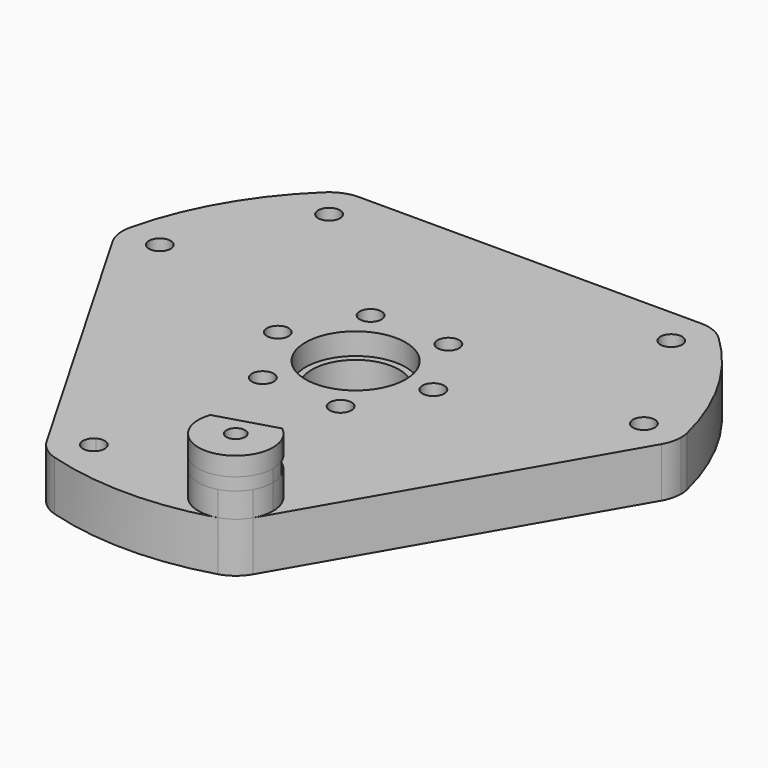
from build123d import *

# Parameters (mm, degrees)
F0_R     = 1.75
F0_R_2   = 8.05
F0_R_3   = 1.5
F0_R_4   = 7
F1_DEPTH = 8
F2_DEPTH = 3.5
F3_DEPTH = 4
F5_DEPTH = 2
F7_DEPTH = 3


# Not quite as in the source:
# - a feature names something its author has since deleted; it is built from what else it names


with BuildPart() as f1:
    # F0 (on Top) → F1 (new body)
    with BuildSketch(Plane.XY):
        with BuildLine():
            ThreePointArc((-32.9057647469, 9.2920110558), (-33.7096123242, 6.2920110558), (-35.9057647469, 4.0958586331))
            Line((-35.9057647469, 4.0958586331), (-14.4057647469, -33.1432337296))
            ThreePointArc((-14.4057647469, -33.1432337296), (-8.4057647469, -33.1432337296), (-5.4057647469, -38.3393861523))
            ThreePointArc((-5.4057647469, -38.3393861523), (-7.8186481903, -43.1490217736), (-13.1166296833, -44.0902940084))
            ThreePointArc((-13.1166296833, -44.0902940084), (-2.42e-07, -46), (13.1166292194, -44.0902941464))
            ThreePointArc((13.1166292194, -44.0902941464), (6.5961292703, -34.7522694018), (17.4057647469, -38.3393861523))
            ThreePointArc((17.4057647469, -38.3393861523), (17.2013197046, -39.892300423), (16.6019171696, -41.3393861523))
            Line((16.6019171696, -41.3393861523), (44.1019171696, 6.2920110558))
            ThreePointArc((44.1019171696, 6.2920110558), (32.9683642938, 10.1564622456), (44.7416293579, 10.685813137))
            ThreePointArc((44.7416293579, 10.685813137), (39.8371685393, 23.0000000602), (31.6250002147, 33.4044811578))
            ThreePointArc((31.6250002147, 33.4044811578), (33.0113519797, 31.4190832059), (33.5, 29.0473750966))
            ThreePointArc((33.5, 29.0473750966), (27.5, 23.0473750966), (21.5, 29.0473750966))
            Line((21.5, 29.0473750966), (-21.5, 29.0473750966))
            ThreePointArc((-21.5, 29.0473750966), (-29.8717083356, 23.5360232142), (-31.624999857, 33.4044814964))
            ThreePointArc((-31.624999857, 33.4044814964), (-39.837168539, 23.0000000607), (-44.7416294721, 10.6858126589))
            ThreePointArc((-44.7416294721, 10.6858126589), (-38.2040484051, 15.2508359547), (-32.9057647469, 9.2920110558))
        make_face()
        with Locations((-6.25, -10.8253175473)):
            Circle(F0_R, mode=Mode.SUBTRACT)
        with Locations((6.25, -10.8253175473)):
            Circle(F0_R, mode=Mode.SUBTRACT)
        with Locations((-12.5, 0)):
            Circle(F0_R, mode=Mode.SUBTRACT)
        with Locations((-6.25, 10.8253175473)):
            Circle(F0_R, mode=Mode.SUBTRACT)
        Circle(F0_R_2, mode=Mode.SUBTRACT)
        with Locations((6.25, 10.8253175473)):
            Circle(F0_R, mode=Mode.SUBTRACT)
        with Locations((12.5, 0)):
            Circle(F0_R, mode=Mode.SUBTRACT)
        with BuildLine():
            Line((27.5, 35.0473750966), (-27.5, 35.0473750966))
            ThreePointArc((-27.5, 35.0473750966), (-23.2573593129, 33.2900157837), (-21.5, 29.0473750966))
            Line((-21.5, 29.0473750966), (21.5, 29.0473750966))
            ThreePointArc((21.5, 29.0473750966), (23.2573593129, 33.2900157837), (27.5, 35.0473750966))
        make_face()
        with BuildLine():
            ThreePointArc((-27.5, 35.0473750966), (-29.7200632424, 34.6215404331), (-31.624999857, 33.4044814964))
            ThreePointArc((-31.624999857, 33.4044814964), (-29.8717083356, 23.5360232142), (-21.5, 29.0473750966))
            ThreePointArc((-21.5, 29.0473750966), (-23.2573593129, 33.2900157837), (-27.5, 35.0473750966))
        make_face()
        with Locations((-27.5, 29.0473750966)):
            Circle(F0_R, mode=Mode.SUBTRACT)
        with BuildLine():
            ThreePointArc((33.5, 29.0473750966), (33.0113519797, 31.4190832059), (31.6250002147, 33.4044811578))
            ThreePointArc((31.6250002147, 33.4044811578), (29.7200634712, 34.621540342), (27.5, 35.0473750966))
            ThreePointArc((27.5, 35.0473750966), (23.2573593129, 33.2900157837), (21.5, 29.0473750966))
            ThreePointArc((21.5, 29.0473750966), (27.5, 23.0473750966), (33.5, 29.0473750966))
        make_face()
        with BuildLine():
            ThreePointArc((29.25, 29.0473750966), (27.5, 27.2973750966), (25.75, 29.0473750966))
            ThreePointArc((25.75, 29.0473750966), (27.5, 30.7973750966), (29.25, 29.0473750966))
        make_face(mode=Mode.SUBTRACT)
        with BuildLine():
            ThreePointArc((44.9057647469, 9.2920110558), (44.864589617, 9.9937276417), (44.7416293579, 10.685813137))
            ThreePointArc((44.7416293579, 10.685813137), (32.9683642938, 10.1564622456), (44.1019171696, 6.2920110558))
            ThreePointArc((44.1019171696, 6.2920110558), (44.7013197046, 7.7390967852), (44.9057647469, 9.2920110558))
        make_face()
        with Locations((38.9057647469, 9.2920110558)):
            Circle(F0_R, mode=Mode.SUBTRACT)
        with BuildLine():
            ThreePointArc((17.4057647469, -38.3393861523), (6.5961292703, -34.7522694018), (13.1166292194, -44.0902941464))
            ThreePointArc((13.1166292194, -44.0902941464), (15.1231017367, -43.049100125), (16.6019171696, -41.3393861523))
            ThreePointArc((16.6019171696, -41.3393861523), (17.2013197046, -39.892300423), (17.4057647469, -38.3393861523))
        make_face()
        with Locations((11.4057647469, -38.3393861523)):
            Circle(F0_R_3, mode=Mode.SUBTRACT)
        with BuildLine():
            ThreePointArc((-5.4057647469, -38.3393861523), (-8.4057647469, -33.1432337296), (-14.4057647469, -33.1432337296))
            ThreePointArc((-14.4057647469, -33.1432337296), (-17.2013197046, -36.7864718817), (-16.6019171696, -41.3393861523))
            ThreePointArc((-16.6019171696, -41.3393861523), (-15.1231019266, -43.0490999751), (-13.1166296833, -44.0902940084))
            ThreePointArc((-13.1166296833, -44.0902940084), (-7.8186481903, -43.1490217736), (-5.4057647469, -38.3393861523))
        make_face()
        with BuildLine():
            ThreePointArc((-9.6557647469, -38.3393861523), (-12.2807647469, -39.854930609), (-12.2807647469, -36.8238416957))
            ThreePointArc((-12.2807647469, -36.8238416957), (-10.5307647469, -36.8238416957), (-9.6557647469, -38.3393861523))
        make_face(mode=Mode.SUBTRACT)
        with BuildLine():
            Line((-14.4057647469, -33.1432337296), (-35.9057647469, 4.0958586331))
            ThreePointArc((-35.9057647469, 4.0958586331), (-40.4586790175, 3.4964560981), (-44.1019171696, 6.2920110558))
            Line((-44.1019171696, 6.2920110558), (-16.6019171696, -41.3393861523))
            ThreePointArc((-16.6019171696, -41.3393861523), (-17.2013197046, -36.7864718817), (-14.4057647469, -33.1432337296))
        make_face()
        with BuildLine():
            ThreePointArc((-44.1019171696, 6.2920110558), (-40.4586790175, 3.4964560981), (-35.9057647469, 4.0958586331))
            ThreePointArc((-35.9057647469, 4.0958586331), (-33.7096123242, 6.2920110558), (-32.9057647469, 9.2920110558))
            ThreePointArc((-32.9057647469, 9.2920110558), (-38.2040484051, 15.2508359547), (-44.7416294721, 10.6858126589))
            ThreePointArc((-44.7416294721, 10.6858126589), (-44.8431651646, 8.4275596228), (-44.1019171696, 6.2920110558))
        make_face()
        with BuildLine():
            ThreePointArc((-38.0307647469, 7.7764665992), (-40.4213092035, 10.1670110558), (-37.1557647469, 9.2920110558))
            ThreePointArc((-37.1557647469, 9.2920110558), (-37.3902202902, 8.4170110558), (-38.0307647469, 7.7764665992))
        make_face(mode=Mode.SUBTRACT)
        Circle(F0_R_2)
        Circle(F0_R_4, mode=Mode.SUBTRACT)
    extrude(amount=-F1_DEPTH)

    # F0 (on Top) → F2 (cut)
    with BuildSketch(Plane.XY):
        Circle(F0_R_2)
        Circle(F0_R_4, mode=Mode.SUBTRACT)
    extrude(amount=-F2_DEPTH, mode=Mode.SUBTRACT)


with BuildPart() as f3:
    # F0 (on Top) → F3 (new body)
    with BuildSketch(Plane.XY):
        with BuildLine():
            ThreePointArc((17.4057647469, -38.3393861523), (6.5961292703, -34.7522694018), (13.1166292194, -44.0902941464))
            ThreePointArc((13.1166292194, -44.0902941464), (15.1231017367, -43.049100125), (16.6019171696, -41.3393861523))
            ThreePointArc((16.6019171696, -41.3393861523), (17.2013197046, -39.892300423), (17.4057647469, -38.3393861523))
        make_face()
        with Locations((11.4057647469, -38.3393861523)):
            Circle(F0_R_3, mode=Mode.SUBTRACT)
    extrude(amount=F3_DEPTH)

    # F4 (on face) → F5 (join)
    with BuildSketch(Plane.XY.offset(4)):
        with BuildLine():
            ThreePointArc((9.9602708355, -38.7400697584), (7.7638146886, -39.2393065877), (5.5427392086, -39.6141141775))
            ThreePointArc((5.5427392086, -39.6141141775), (12.0467978079, -44.3050442564), (17.4057647469, -38.3393861523))
            ThreePointArc((17.4057647469, -38.3393861523), (17.3065432967, -37.2527341815), (17.0121605783, -36.2020219388))
            ThreePointArc((17.0121605783, -36.2020219388), (14.947389292, -37.1022311102), (12.8352193016, -37.8847877845))
            ThreePointArc((12.8352193016, -37.8847877845), (12.8880234679, -38.1093664054), (12.9057647469, -38.3393861523))
            ThreePointArc((12.9057647469, -38.3393861523), (11.607951706, -39.8256971674), (9.9602708355, -38.7400697584))
        make_face()
    extrude(amount=F5_DEPTH)

    # F6 (on face) → F7 (join)
    with BuildSketch(Plane.XY.offset(6)):
        with BuildLine():
            ThreePointArc((5.5427392086, -39.6141141775), (13.1166294589, -44.0902940752), (17.0121605783, -36.2020219388))
            ThreePointArc((17.0121605783, -36.2020219388), (14.947389292, -37.1022311102), (12.8352193016, -37.8847877845))
            ThreePointArc((12.8352193016, -37.8847877845), (12.8880234679, -38.1093664054), (12.9057647469, -38.3393861523))
            ThreePointArc((12.9057647469, -38.3393861523), (11.607951706, -39.8256971674), (9.9602708355, -38.7400697584))
            ThreePointArc((9.9602708355, -38.7400697584), (7.7638146886, -39.2393065877), (5.5427392086, -39.6141141775))
        make_face()
        with BuildLine():
            ThreePointArc((12.8352193016, -37.8847877845), (14.947389292, -37.1022311102), (17.0121605783, -36.2020219388))
            ThreePointArc((17.0121605783, -36.2020219388), (16.2239290423, -34.7637333696), (15.0756758433, -33.5926238301))
            Line((15.0756758433, -33.5926238301), (5.737994077, -36.3705348035))
            ThreePointArc((5.737994077, -36.3705348035), (5.4166064515, -37.9788547209), (5.5427392086, -39.6141141775))
            ThreePointArc((5.5427392086, -39.6141141775), (7.7638146886, -39.2393065877), (9.9602708355, -38.7400697584))
            ThreePointArc((9.9602708355, -38.7400697584), (10.9780485689, -36.9016591716), (12.8352193016, -37.8847877845))
        make_face()
    extrude(amount=F7_DEPTH)


solid = Compound([f1.part, f3.part])
